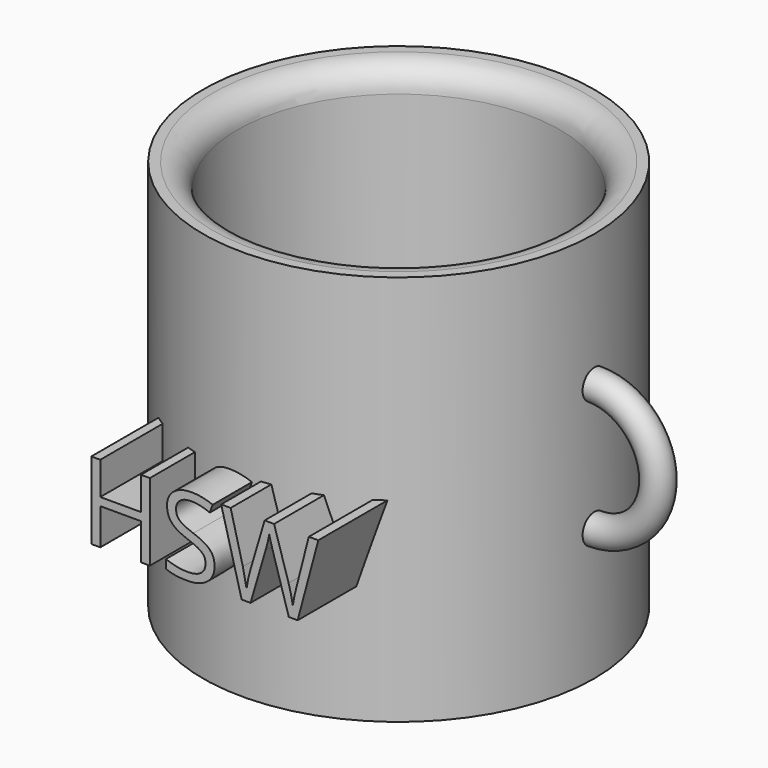
from build123d import *

# Parameters (mm, degrees)
F2_R          = 3
F3_ANGLE_BACK = 90
F3_ANGLE      = 180
F5_TEXT_SIZE  = 22.0872446162


# Not quite as in the source:
# - Text() gives the source's letters only with a copy of the font that has no kerning and outlines rounded to 1/6400 em; it was checked with that copy


with BuildPart() as f1:
    # F0 (on Front) → F1 (revolve)
    with BuildSketch(Plane.XZ):
        with BuildLine():
            Line((40, 40), (38.0249720588, 40))
            ThreePointArc((38.0249720588, 40), (34.4894381529, 38.5355339059), (33.0249720588, 35))
            Line((33.0249720588, 35), (33.0249720588, -37))
            Line((33.0249720588, -37), (0, -37))
            Line((0, -37), (0, -40))
            Line((0, -40), (40, -40))
            Line((40, -40), (40, 40))
        make_face()
    revolve(axis=Axis((0, 0, 0), (0, 0, -1)))


with BuildPart() as f3:
    # F2 (on Top) → F3 (revolve)
    with BuildSketch(Plane.XY, mode=Mode.PRIVATE) as f3_sk:
        with Locations((53, 0)):
            Circle(F2_R)
    revolve(f3_sk.sketch.rotate(Axis((40, -2.4495963007, 0), (0, 1, 0)), -F3_ANGLE_BACK), axis=Axis((40, -2.4495963007, 0), (0, 1, 0)), revolution_arc=F3_ANGLE)


with BuildPart() as f6:
    # F5 (on offset) → F6 (new body, up to the next surface of F1)
    with BuildSketch(Plane.XZ.offset(50)):
        with Locations((-25, -15.9028161237)):
            Text('HSW', F5_TEXT_SIZE, font='Open Sans', text_align=(TextAlign.LEFT, TextAlign.BOTTOM))
    extrude(until=Until.NEXT, target=f1.part, dir=(0, 1, 0))


solid = Compound([f1.part, f3.part, f6.part])
